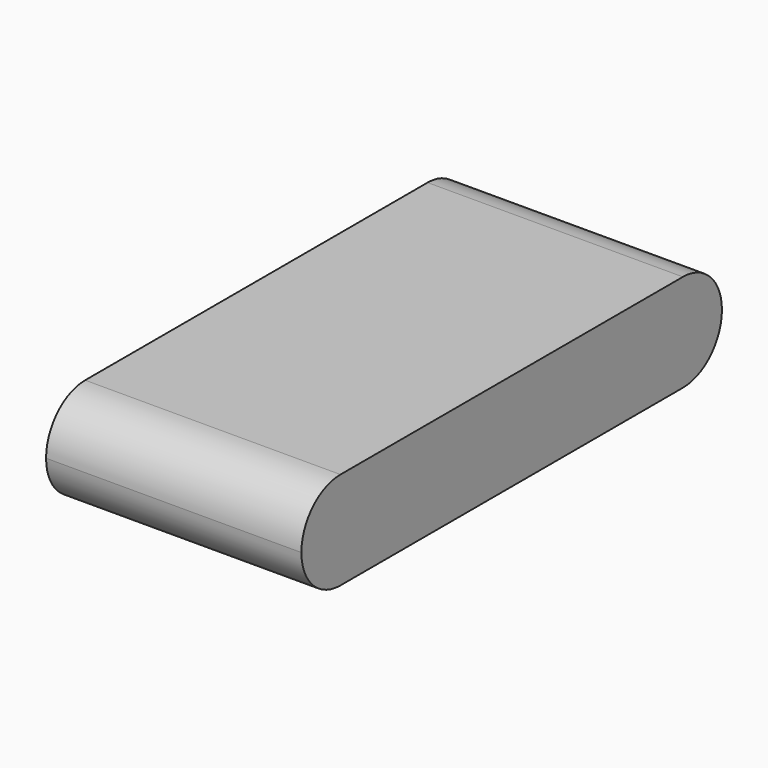
from build123d import *

# Parameters (mm, degrees)
F0_W     = 34
F0_H     = 70
F1_DEPTH = 13
F2_R     = 6.49999
F3_R     = 6.49999


# Not quite as in the source:
# - a fillet or chamfer is up to 0.001 mm smaller than in the source, because OpenCascade refuses the exact size


with BuildPart() as f1:
    # F0 (on Top) → F1 (new body)
    with BuildSketch(Plane.XY):
        with Locations((17, 35)):
            Rectangle(F0_W, F0_H)
    extrude(amount=F1_DEPTH)

    # F2 (radius 6.5 in the source; OpenCascade refuses exactly that, so slightly less here)
    f2_edges = [f1.edges().sort_by_distance(p)[0] for p in [
        (17, 0, 13),
        (17, 0, 0),
    ]]
    fillet(f2_edges, radius=F2_R)

    # F3 (radius 6.5 in the source; OpenCascade refuses exactly that, so slightly less here)
    f3_edges = [f1.edges().sort_by_distance(p)[0] for p in [
        (17, 70, 13),
        (17, 70, 0),
    ]]
    fillet(f3_edges, radius=F3_R)


solid = f1.part
